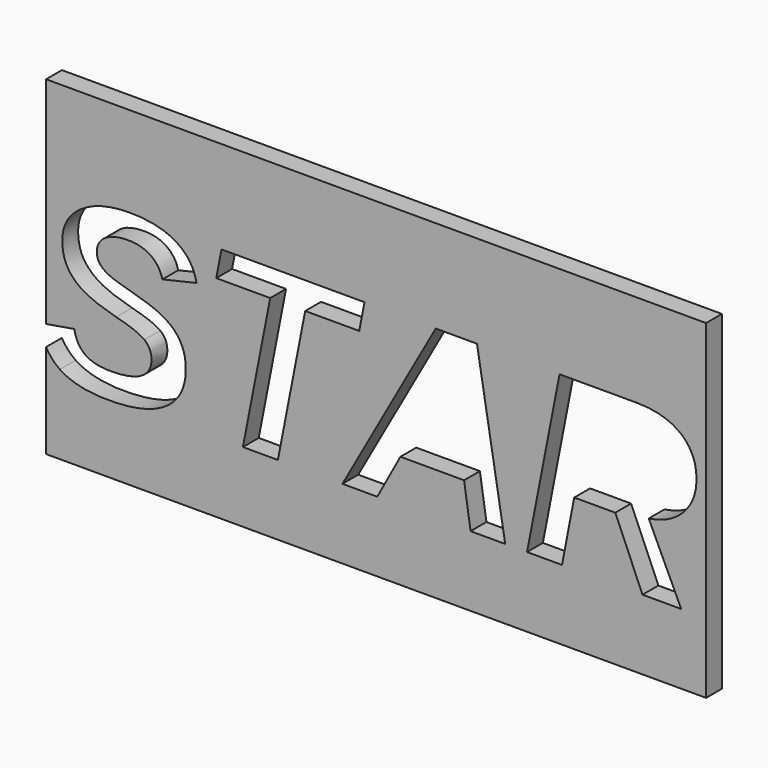
from build123d import *

# Parameters (mm, degrees)
F1_DEPTH = 3


with BuildPart() as f1:
    # F0 (on Front) → F1 (new body)
    with BuildSketch(Plane.XZ):
        with BuildLine():
            Line((-100, 0), (0, 0))
            Line((0, 0), (0, 50))
            Line((0, 50), (-100, 50))
            Line((-100, 50), (-100, 17.3523504695))
            Line((-100, 17.3523504695), (-95.7282808558, 18.0761301251))
            add(Edge.make_bspline(
                [(-95.7282808558, 18.0761301251), (-95.3488123547, 16.081045733), (-94.0465454532, 15.1639968553)],
                knots=[0, 0, 0, 1, 1, 1], degree=2))
            add(Edge.make_bspline(
                [(-94.0465454532, 15.1639968553), (-92.7442785517, 14.2469479777), (-90.2259875899, 14.2469479777)],
                knots=[0, 0, 0, 1, 1, 1], degree=2))
            add(Edge.make_bspline(
                [(-90.2259875899, 14.2469479777), (-84.0280020719, 14.2469479777), (-84.0280020719, 17.8231511244)],
                knots=[0, 0, 0, 1, 1, 1], degree=2))
            add(Edge.make_bspline(
                [(-84.0280020719, 17.8231511244), (-84.0280020719, 19.2605318104), (-85.1060375864, 20.0970873696)],
                knots=[0, 0, 0, 1, 1, 1], degree=2))
            add(Edge.make_bspline(
                [(-85.1060375864, 20.0970873696), (-86.1840731009, 20.9336429289), (-89.3865572693, 21.738576113)],
                knots=[0, 0, 0, 1, 1, 1], degree=2))
            add(Edge.make_bspline(
                [(-89.3865572693, 21.738576113), (-92.692532847, 22.6182530928), (-94.2822758857, 23.5726738683)],
                knots=[0, 0, 0, 1, 1, 1], degree=2))
            add(Edge.make_bspline(
                [(-94.2822758857, 23.5726738683), (-95.8720189244, 24.5270946438), (-96.7056997223, 25.9012305796)],
                knots=[0, 0, 0, 1, 1, 1], degree=2))
            add(Edge.make_bspline(
                [(-96.7056997223, 25.9012305796), (-97.5393805202, 27.2753665154), (-97.5393805202, 29.2704509076)],
                knots=[0, 0, 0, 1, 1, 1], degree=2))
            add(Edge.make_bspline(
                [(-97.5393805202, 29.2704509076), (-97.5393805202, 32.449936985), (-94.7192396143, 34.390400911)],
                knots=[0, 0, 0, 1, 1, 1], degree=2))
            add(Edge.make_bspline(
                [(-94.7192396143, 34.390400911), (-91.8990987084, 36.3308648371), (-87.2477348085, 36.3308648371)],
                knots=[0, 0, 0, 1, 1, 1], degree=2))
            add(Edge.make_bspline(
                [(-87.2477348085, 36.3308648371), (-82.9700898871, 36.3308648371), (-80.3828046523, 34.7756189349)],
                knots=[0, 0, 0, 1, 1, 1], degree=2))
            add(Edge.make_bspline(
                [(-80.3828046523, 34.7756189349), (-77.7955194175, 33.2203730326), (-77.2033185749, 30.2363707285)],
                knots=[0, 0, 0, 1, 1, 1], degree=2))
            Line((-77.2033185749, 30.2363707285), (-82.3778890444, 29.0347204751))
            add(Edge.make_bspline(
                [(-82.3778890444, 29.0347204751), (-82.7746061138, 30.6503363661), (-84.0941215835, 31.6133814257)],
                knots=[0, 0, 0, 1, 1, 1], degree=2))
            add(Edge.make_bspline(
                [(-84.0941215835, 31.6133814257), (-85.4136370532, 32.5764264853), (-87.5352109457, 32.5764264853)],
                knots=[0, 0, 0, 1, 1, 1], degree=2))
            add(Edge.make_bspline(
                [(-87.5352109457, 32.5764264853), (-89.7602762476, 32.5764264853), (-91.0366702968, 31.7398709261)],
                knots=[0, 0, 0, 1, 1, 1], degree=2))
            add(Edge.make_bspline(
                [(-91.0366702968, 31.7398709261), (-92.3130643459, 30.9033153668), (-92.3130643459, 29.4486861126)],
                knots=[0, 0, 0, 1, 1, 1], degree=2))
            add(Edge.make_bspline(
                [(-92.3130643459, 29.4486861126), (-92.3130643459, 28.6035062693), (-91.8444782423, 28.0113054266)],
                knots=[0, 0, 0, 1, 1, 1], degree=2))
            add(Edge.make_bspline(
                [(-91.8444782423, 28.0113054266), (-91.3758921387, 27.419104584), (-90.4789665906, 26.9792660941)],
                knots=[0, 0, 0, 1, 1, 1], degree=2))
            add(Edge.make_bspline(
                [(-90.4789665906, 26.9792660941), (-89.5820410426, 26.5394276042), (-86.9200120121, 25.8207372612)],
                knots=[0, 0, 0, 1, 1, 1], degree=2))
            add(Edge.make_bspline(
                [(-86.9200120121, 25.8207372612), (-84.0682487312, 25.0273031225), (-82.7027370795, 24.3373603933)],
                knots=[0, 0, 0, 1, 1, 1], degree=2))
            add(Edge.make_bspline(
                [(-82.7027370795, 24.3373603933), (-81.3372254278, 23.647417664), (-80.5179184368, 22.7849892524)],
                knots=[0, 0, 0, 1, 1, 1], degree=2))
            add(Edge.make_bspline(
                [(-80.5179184368, 22.7849892524), (-79.6986114458, 21.9225608408), (-79.26739724, 20.8071534285)],
                knots=[0, 0, 0, 1, 1, 1], degree=2))
            add(Edge.make_bspline(
                [(-79.26739724, 20.8071534285), (-78.8361830342, 19.6917460162), (-78.8361830342, 18.237116762)],
                knots=[0, 0, 0, 1, 1, 1], degree=2))
            add(Edge.make_bspline(
                [(-78.8361830342, 18.237116762), (-78.8361830342, 14.3561889098), (-81.8201853383, 12.3151083357)],
                knots=[0, 0, 0, 1, 1, 1], degree=2))
            add(Edge.make_bspline(
                [(-81.8201853383, 12.3151083357), (-84.8041876424, 10.2740277616), (-90.5882075228, 10.2740277616)],
                knots=[0, 0, 0, 1, 1, 1], degree=2))
            add(Edge.make_bspline(
                [(-90.5882075228, 10.2740277616), (-95.3833094912, 10.2740277616), (-97.8987256917, 11.9730117325)],
                knots=[0, 0, 0, 1, 1, 1], degree=2))
            add(Edge.make_bspline(
                [(-97.8987256917, 11.9730117325), (-99.2313673487, 12.8731159831), (-100, 14.2855889299)],
                knots=[0, 0, 0, 0.529789725, 0.529789725, 0.529789725], degree=2))
            Line((-100, 14.2855889299), (-100, 0))
        make_face()
        Polygon((-52.5493650489, 31.8577361423), (-60.742434959, 31.8577361423), (-64.8763418119, 10.6362476945), (-70.1774017818, 10.6362476945), (-66.0434949289, 31.8577361423), (-74.2193162708, 31.8577361423), (-73.4258821321, 35.951396336), (-51.761680433, 35.951396336), align=None, mode=Mode.SUBTRACT)
        Polygon((-30.4367005758, 10.6362476945), (-35.6802653183, 10.6362476945), (-36.6691832302, 17.1044607814), (-46.3168823945, 17.1044607814), (-49.8183417456, 10.6362476945), (-55.1021531472, 10.6362476945), (-40.9640767199, 35.951396336), (-34.7085959745, 35.951396336), align=None, mode=Mode.SUBTRACT)
        with BuildLine():
            Line((-3.7704140895, 10.6362476945), (-9.6291777655, 10.6362476945))
            Line((-9.6291777655, 10.6362476945), (-13.7573350957, 20.2322011541))
            Line((-13.7573350957, 20.2322011541), (-19.9783187046, 20.2322011541))
            Line((-19.9783187046, 20.2322011541), (-21.8296650281, 10.6362476945))
            Line((-21.8296650281, 10.6362476945), (-27.1249754753, 10.6362476945))
            Line((-27.1249754753, 10.6362476945), (-22.2033840065, 35.951396336))
            Line((-22.2033840065, 35.951396336), (-10.5088547453, 35.951396336))
            add(Edge.make_bspline(
                [(-10.5088547453, 35.951396336), (-7.6513419416, 35.951396336), (-5.6131361289, 35.0717193562)],
                knots=[0, 0, 0, 1, 1, 1], degree=2))
            add(Edge.make_bspline(
                [(-5.6131361289, 35.0717193562), (-3.5749303162, 34.1920423764), (-2.5141433699, 32.5563031557)],
                knots=[0, 0, 0, 1, 1, 1], degree=2))
            add(Edge.make_bspline(
                [(-2.5141433699, 32.5563031557), (-1.4533564237, 30.9205639351), (-1.4533564237, 28.7127472014)],
                knots=[0, 0, 0, 1, 1, 1], degree=2))
            add(Edge.make_bspline(
                [(-1.4533564237, 28.7127472014), (-1.4533564237, 25.7459934655), (-3.4024446338, 23.6790400391)],
                knots=[0, 0, 0, 1, 1, 1], degree=2))
            add(Edge.make_bspline(
                [(-3.4024446338, 23.6790400391), (-5.351532844, 21.6120866127), (-8.6920055583, 21.1118781339)],
                knots=[0, 0, 0, 1, 1, 1], degree=2))
            Line((-8.6920055583, 21.1118781339), (-3.7704140895, 10.6362476945))
        make_face(mode=Mode.SUBTRACT)
    extrude(amount=F1_DEPTH)


solid = f1.part
